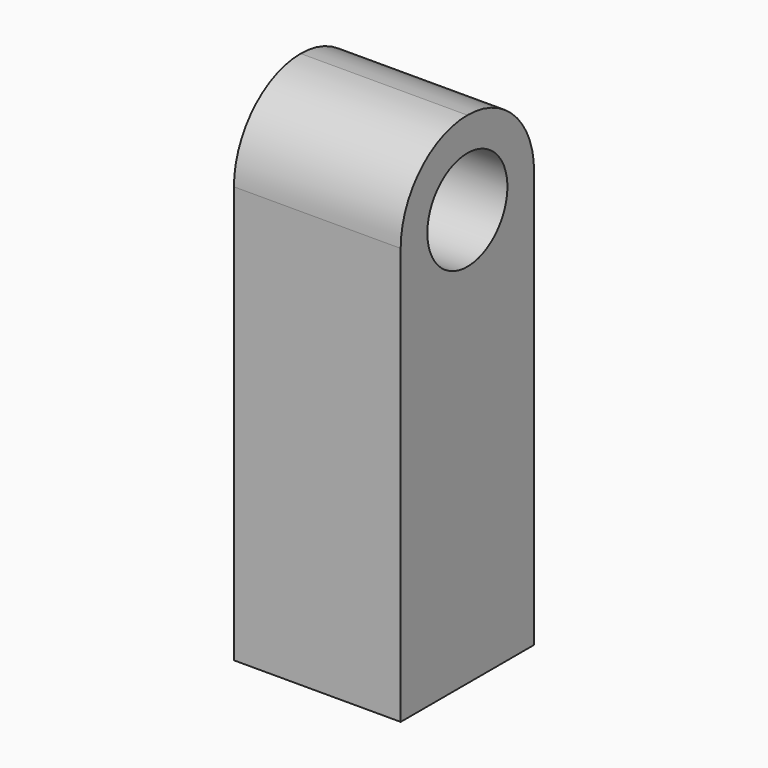
from build123d import *

# Parameters (mm, degrees)
F0_W     = 10
F0_H     = 10
F1_DEPTH = 20
F2_W     = 2
F2_H     = 10
F2_W_2   = 10
F3_DEPTH = 10
F6_R     = 4.99999
F5_W     = 10
F5_H     = 10
F5_R     = 3
F7_DEPTH = 2
F4_W     = 10
F4_H     = 10
F4_R     = 3
F8_DEPTH = 2
F9_DEPTH = 14.001


# Not quite as in the source:
# - a fillet or chamfer is up to 0.001 mm smaller than in the source, because OpenCascade refuses the exact size


with BuildPart() as f1:
    # F0 (on Top) → F1 (new body)
    with BuildSketch(Plane.XY):
        Rectangle(F0_W, F0_H)
    extrude(amount=F1_DEPTH)

    # F2 (on face) → F3 (join)
    with BuildSketch(Plane.XY.offset(20)):
        with Locations((-6, 0)):
            Rectangle(F2_W, F2_H)
        Rectangle(F2_W_2, F2_H)
        with Locations((6, 0)):
            Rectangle(F2_W, F2_H)
    extrude(amount=F3_DEPTH)

    # F6 (radius 5 in the source; OpenCascade refuses exactly that, so slightly less here)
    f6_edges = [f1.edges().sort_by_distance(p)[0] for p in [
        (0, 5, 30),
        (0, -5, 30),
    ]]
    fillet(f6_edges, radius=F6_R)

    # F5 (on face) → F7 (cut)
    with BuildSketch(Plane.YZ.offset(7)):
        with Locations((0, 25)):
            Rectangle(F5_W, F5_H)
        with Locations((0, 25)):
            Circle(F5_R, mode=Mode.SUBTRACT)
    extrude(amount=-F7_DEPTH, mode=Mode.SUBTRACT)

    # F4 (on face) → F8 (cut)
    with BuildSketch(Plane(origin=(-7, 0, 0), x_dir=(0, -1, 0), z_dir=(-1, 0, 0))):
        with Locations((0, 25)):
            Rectangle(F4_W, F4_H)
        with Locations((0, 25)):
            Circle(F4_R, mode=Mode.SUBTRACT)
    extrude(amount=-F8_DEPTH, mode=Mode.SUBTRACT)

    # F9 (cut, through all): a face of the model
    f9_faces = [f1.faces().sort_by_distance(p)[0] for p in [
        (-7, 0, 25),
    ]]
    extrude(f9_faces, amount=-F9_DEPTH, mode=Mode.SUBTRACT)


solid = f1.part
